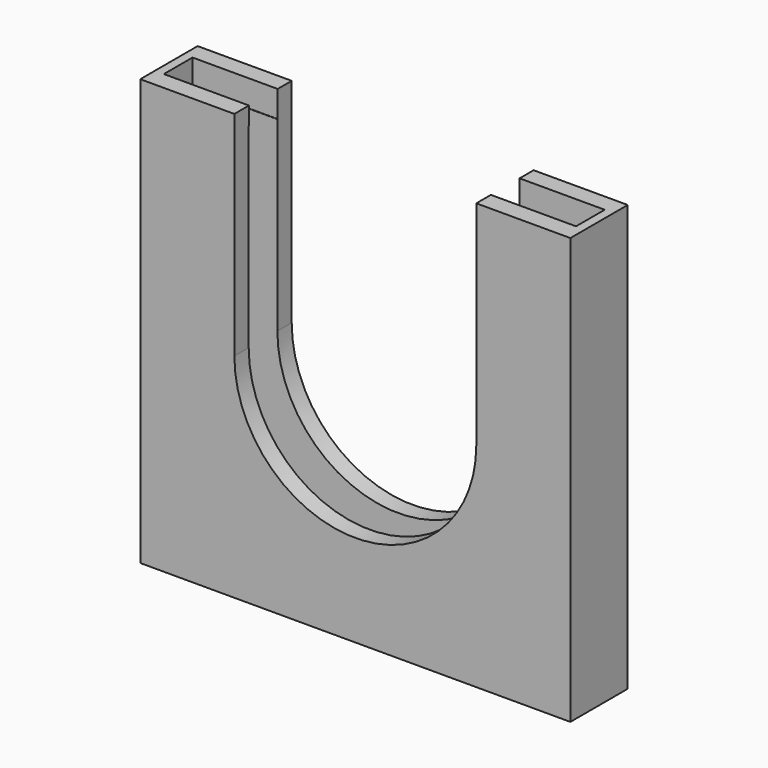
from build123d import *

# Parameters (mm, degrees)
F1_DEPTH = 50.8
F2_T     = -12.7
F3_W     = 25.4
F3_H     = 38.1000075253
F4_DEPTH = 146.05
F5_DEPTH = 146.05


with BuildPart() as f1:
    # F0 (on Front) → F1 (new body)
    with BuildSketch(Plane.XZ):
        with BuildLine():
            Line((152.4, -150.9333811935), (152.4, 150.9333811935))
            Line((152.4, 150.9333811935), (85.725, 150.9333811935))
            Line((85.725, 150.9333811935), (85.725, 0))
            ThreePointArc((85.725, 0), (0, -85.725), (-85.725, 0))
            Line((-85.725, 0), (-85.725, 150.9333811935))
            Line((-85.725, 150.9333811935), (-152.4, 150.9333811935))
            Line((-152.4, 150.9333811935), (-152.4, -150.9333811935))
            Line((-152.4, -150.9333811935), (152.4, -150.9333811935))
        make_face()
    extrude(amount=F1_DEPTH)

    # F2
    f2_openings = [f1.faces().sort_by_distance(p)[0] for p in [
        (85.725, -25.4, 75.466691),
        (0, -25.4, -85.725),
        (-85.725, -25.4, 75.466691),
    ]]
    offset(amount=F2_T, openings=f2_openings)

    # F3 (on Right) → F4 (cut)
    with BuildSketch(Plane.YZ):
        with Locations((-25.1512676477, 151.2203067541)):
            Rectangle(F3_W, F3_H)
    extrude(amount=-F4_DEPTH, mode=Mode.SUBTRACT)

    # F3 (on Right) → F5 (cut)
    with BuildSketch(Plane.YZ):
        with Locations((-25.1512676477, 151.2203067541)):
            Rectangle(F3_W, F3_H)
    extrude(amount=F5_DEPTH, mode=Mode.SUBTRACT)


solid = f1.part
